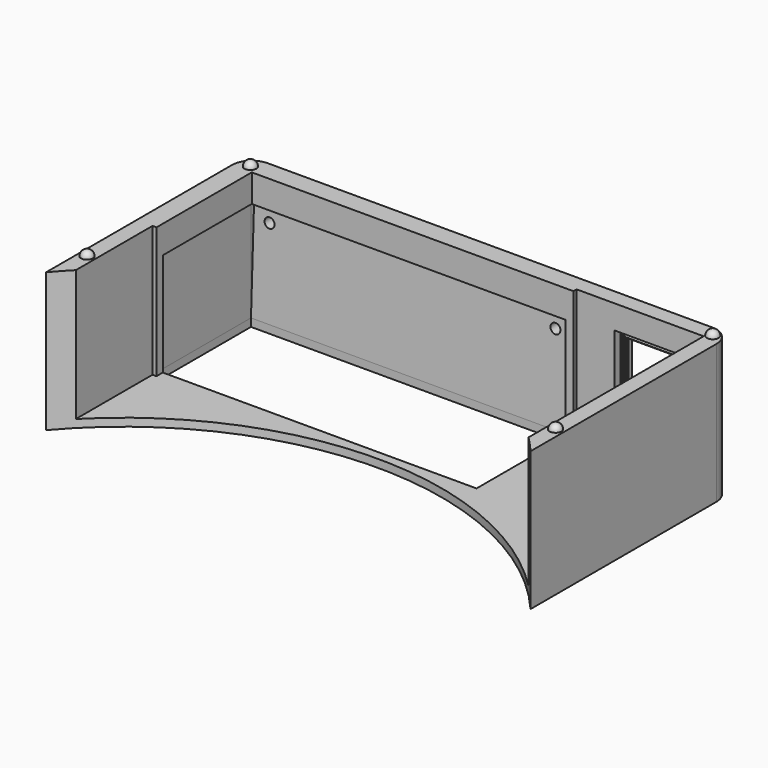
from build123d import *
from build123d import SkipClean  # not in build123d's __all__

# Parameters (mm, degrees)
F0_W       = 122
F0_H       = 63.5
F1_DEPTH   = 35
F2_W       = 114.0000007153
F2_H       = 55.5000007153
F3_DEPTH   = 33
F4_W       = 80
F4_H       = 29
F5_DEPTH   = 35.001
F6_W       = 80.0000003576
F6_H       = 7
F7_DEPTH   = 1
F8_W       = 80
F8_H       = 26
F9_DEPTH   = 1
F11_DEPTH  = 80
F13_DEPTH  = 1
F14_R      = 80
F15_DEPTH  = 35.001
F17_D      = 2.5
F18_W      = 17
F18_H      = 23
F19_DEPTH  = 2
F20_W      = 15.9999973774
F20_H      = 21.9999973774
F21_DEPTH  = 0.6
F21_TAPER  = 59
F22_DEPTH  = 0.6
F23_W      = 13.0028597713
F23_H      = 19.0028597713
F24_DEPTH  = 1
F24_FACE_W = 13.0028597713
F24_FACE_H = 19.0028597713
F25_DEPTH  = 1
F25_TAPER  = -45
F26_R      = 5
F27_R      = 1.5
F28_DEPTH  = 1.5
F29_R      = 1.49999


# Not quite as in the source:
# - a fillet or chamfer is up to 0.001 mm smaller than in the source, because OpenCascade refuses the exact size
# - ends of sketch curves that miss each other by under 0.0002 mm in the source are joined


with BuildPart() as f1:
    # F0 (on Top) → F1 (new body)
    with BuildSketch(Plane.XY):
        Rectangle(F0_W, F0_H)
    extrude(amount=F1_DEPTH)

    # F2 (on face) → F3 (cut)
    with BuildSketch(Plane.XY.offset(35)):
        Rectangle(F2_W, F2_H)
    extrude(amount=-F3_DEPTH, mode=Mode.SUBTRACT)

    # F4 (on face) → F5 (cut, through all)
    with BuildSketch(Plane(origin=(0, 0, 0), x_dir=(1, 0, 0), z_dir=(0, 0, -1))):
        with Locations((-17, -13.25)):
            Rectangle(F4_W, F4_H)
    with SkipClean():  # cleaning this boolean's faces spoils the solid; the shape is the same uncleaned
        extrude(amount=-F5_DEPTH, mode=Mode.SUBTRACT)

    # F6 (on face) → F7 (join)
    with BuildSketch(Plane.XZ.offset(-27.7500003576)):
        Polygon((23, 28), (23, 2), (25, 2), (25, 35), (23, 35), align=None)
        with Locations((-17.0000001788, 31.5)):
            Rectangle(F6_W, F6_H)
    extrude(amount=F7_DEPTH)

    # F8 (on face) → F9 (cut)
    with BuildSketch(Plane.XZ.offset(-27.7500003576)):
        with Locations((-17, 15)):
            Rectangle(F8_W, F8_H)
    extrude(amount=-F9_DEPTH, mode=Mode.SUBTRACT)

    # F10 (on face) → F11 (join, through all)
    with BuildSketch(Plane(origin=(23, 0, 0), x_dir=(0, -1, 0), z_dir=(-1, 0, 0))):
        Polygon((-28.7500003576, 2), (-27.7500003576, 2), (-28.7500003576, 28), align=None)
    extrude(amount=F11_DEPTH)

    # F12 (on face) → F13 (join)
    with BuildSketch(Plane.YZ.offset(-57.0000003576)):
        Polygon((-3.25, 2), (-1.25, 2), (-1.25, 28), (26.7500003576, 28), (26.7500003576, 35), (-1.25, 35), (-3.25, 35), align=None)
    extrude(amount=F13_DEPTH)

    # F14 (on face) → F15 (cut, through all)
    with BuildSketch(Plane(origin=(0, 0, 0), x_dir=(1, 0, 0), z_dir=(0, 0, -1))):
        with Locations((0, 83.5090571784)):
            Circle(F14_R)
        with BuildLine():
            Line((61, 31.75), (-61, 31.75))
            ThreePointArc((-61, 31.75), (0, 3.5090571784), (61, 31.75))
        make_face()
    extrude(amount=-F15_DEPTH, mode=Mode.SUBTRACT)

    # F17 (through all)
    with Locations(Plane(origin=(0, 31.75, 0), x_dir=(-1, 0, 0), z_dir=(0, 1, 0))):
        with Locations((-19, 24), (53, 24)):
            Hole(F17_D / 2)

    # F18 (on face) → F19 (cut)
    with BuildSketch(Plane.XZ.offset(-27.7500003576)):
        with Locations((43.0000003576, 17.5)):
            Rectangle(F18_W, F18_H)
    extrude(amount=-F19_DEPTH, mode=Mode.SUBTRACT)

    # F20 (on face) → F21 (join)
    with BuildSketch(Plane.XZ.offset(-29.7500003576)):
        with Locations((43.0000003576, 17.5)):
            Rectangle(F20_W, F20_H)
    extrude(amount=F21_DEPTH, taper=F21_TAPER)

    # F22 (cut): a face of the model
    f22_faces = [f1.faces().sort_by_distance(p)[0] for p in [
        (43.0000003576, 29.1500003576, 17.5),
    ]]
    extrude(f22_faces, amount=-F22_DEPTH, mode=Mode.SUBTRACT)

    # F23 (on face) → F24 (cut)
    with BuildSketch(Plane.XZ.offset(-29.7500003576)):
        with Locations((43.0000003576, 17.5)):
            Rectangle(F23_W, F23_H)
    extrude(amount=-F24_DEPTH, mode=Mode.SUBTRACT)

    # F24_face (on face) → F25 (cut)
    with BuildSketch(Plane(origin=(43.0000003576, 30.7500003576, 17.5), x_dir=(1, 0, 0), z_dir=(0, -1, 0))):
        Rectangle(F24_FACE_W, F24_FACE_H)
    extrude(amount=-F25_DEPTH, taper=F25_TAPER, mode=Mode.SUBTRACT)

    # F26
    f26_edges = [f1.edges().sort_by_distance(p)[0] for p in [
        (61, 31.75, 17.5),
        (-61, 31.75, 17.5),
    ]]
    fillet(f26_edges, radius=F26_R)

    # F27 (on face) → F28 (join)
    with BuildSketch(Plane.XY.offset(35)):
        with Locations((58.2677671318, 29.0177671318)):
            Circle(F27_R)
        with Locations((59.0000001788, -21.3752887388)):
            Circle(F27_R)
        with Locations((-59.0000001788, -21.3752887388)):
            Circle(F27_R)
        with Locations((-57.7677671318, 28.5177671318)):
            Circle(F27_R)
    extrude(amount=F28_DEPTH)

    # F29 (radius 1.5 in the source; OpenCascade refuses exactly that, so slightly less here)
    f29_edges = [f1.edges().sort_by_distance(p)[0] for p in [
        (57.5, -21.375289, 36.5),
        (-60.5, -21.375289, 36.5),
        (-59.267767, 28.517767, 36.5),
        (56.767767, 29.017767, 36.5),
    ]]
    fillet(f29_edges, radius=F29_R)


solid = f1.part
